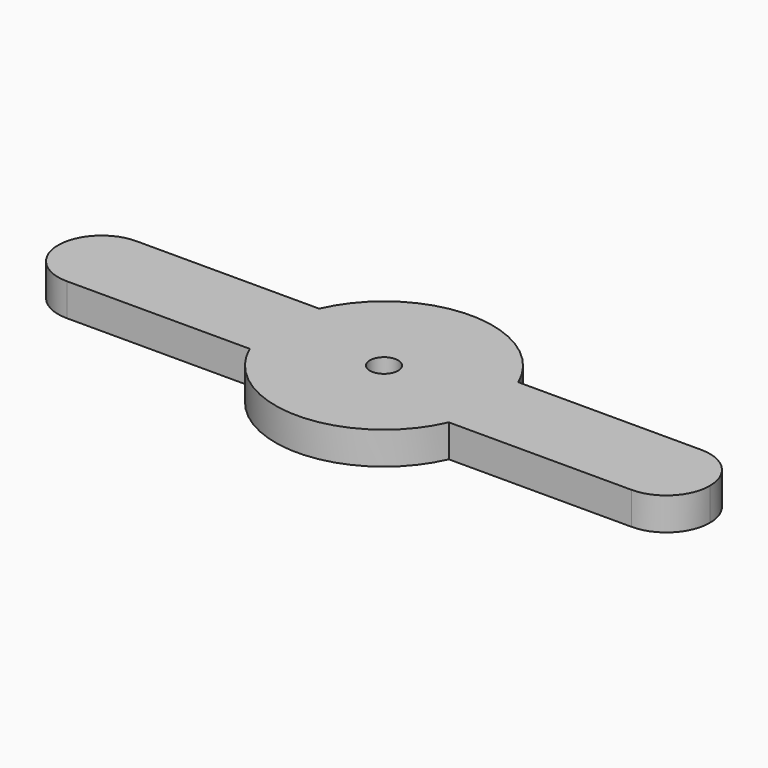
from build123d import *

# Parameters (mm, degrees)
F2_W      = 60
F2_H      = 8
F2_R      = 3
F4_DEPTH  = 4
F5_R      = 3.99999
F6_R      = 10
F7_DEPTH  = 3
F3_R      = 1.3
F8_DEPTH  = 4.001
F9_W      = 25
F9_H      = 8
F10_DEPTH = 1
F11_DEPTH = 2


# Not quite as in the source:
# - a fillet or chamfer is up to 0.001 mm smaller than in the source, because OpenCascade refuses the exact size


with BuildPart() as f4:
    # F2 (on face) → F4 (new body)
    with BuildSketch(Plane.XY):
        with Locations((0, 38)):
            Rectangle(F2_W, F2_H)
        with Locations((-26, 38)):
            Circle(F2_R, mode=Mode.SUBTRACT)
        Polygon((1.1402667816, 36.025), (0, 36.025), (-1.1402667816, 36.025), (-2.2805335633, 38), (-1.1402667816, 39.975), (0, 39.975), (1.1402667816, 39.975), (2.2805335633, 38), align=None, mode=Mode.SUBTRACT)
        with Locations((26, 38)):
            Circle(F2_R, mode=Mode.SUBTRACT)
        Polygon((-1.1402667816, 36.025), (0, 36.025), (1.1402667816, 36.025), (2.2805335633, 38), (1.1402667816, 39.975), (0, 39.975), (-1.1402667816, 39.975), (-2.2805335633, 38), align=None)
        with Locations((-26, 38)):
            Circle(F2_R)
        with Locations((26, 38)):
            Circle(F2_R)
    extrude(amount=F4_DEPTH)

    # F5 (radius 4 in the source; OpenCascade refuses exactly that, so slightly less here)
    f5_edges = [f4.edges().sort_by_distance(p)[0] for p in [
        (-30, 42, 2),
        (-30, 34, 2),
        (30, 42, 2),
        (30, 34, 2),
    ]]
    fillet(f5_edges, radius=F5_R)

    # F6 (on face) → F7 (join)
    with BuildSketch(Plane.XY.offset(4)):
        with Locations((0, 38)):
            Circle(F6_R)
    extrude(amount=-F7_DEPTH)

    # F3 (on face) → F8 (cut, through all)
    with BuildSketch(Plane.XY):
        with Locations((0, 38)):
            Circle(F3_R)
    extrude(amount=F8_DEPTH, mode=Mode.SUBTRACT)

    # F9 (on face) → F10 (cut)
    with BuildSketch(Plane.XY):
        with Locations((17.5, 38)):
            Rectangle(F9_W, F9_H)
        with Locations((-17.5, 38)):
            Rectangle(F9_W, F9_H)
    extrude(amount=F10_DEPTH, mode=Mode.SUBTRACT)

    # F2 (on face) → F11 (cut)
    with BuildSketch(Plane.XY):
        Polygon((-1.1402667816, 36.025), (0, 36.025), (1.1402667816, 36.025), (2.2805335633, 38), (1.1402667816, 39.975), (0, 39.975), (-1.1402667816, 39.975), (-2.2805335633, 38), align=None)
    extrude(amount=F11_DEPTH, mode=Mode.SUBTRACT)


solid = f4.part
